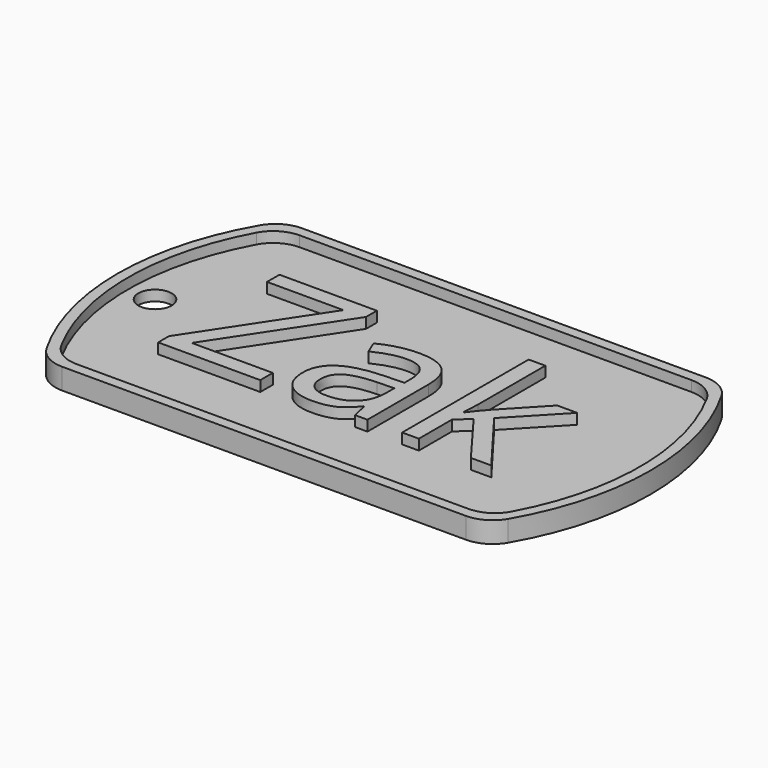
from build123d import *

# Parameters (mm, degrees)
F1_DEPTH     = 1
F3_DEPTH     = 1
F4_R         = 1.5875
F5_DEPTH     = 1
F6_TEXT_SIZE = 19.8251166795
F7_DEPTH     = 1


# Not quite as in the source:
# - a feature of the source that left no trace in its solid (it failed there, or was rolled back) is left out
# - Text() gives the source's letters only with a copy of the font that has no kerning and outlines rounded to 1/6400 em; it was checked with that copy


with BuildPart() as f1:
    # F0 (on Top) → F1 (new body)
    with BuildSketch(Plane.XY):
        with BuildLine():
            ThreePointArc((-19.2474145991, 14.2875), (-20.8349145991, 13.862130657), (-21.9970452561, 12.7))
            ThreePointArc((-21.9970452561, 12.7), (-25.4, 0), (-21.9970452561, -12.7))
            ThreePointArc((-21.9970452561, -12.7), (-20.8349145991, -13.862130657), (-19.2474145991, -14.2875))
            Line((-19.2474145991, -14.2875), (19.2474145991, -14.2875))
            ThreePointArc((19.2474145991, -14.2875), (20.8349145991, -13.862130657), (21.9970452561, -12.7))
            ThreePointArc((21.9970452561, -12.7), (25.4, 0), (21.9970452561, 12.7))
            ThreePointArc((21.9970452561, 12.7), (20.8349145991, 13.862130657), (19.2474145991, 14.2875))
            Line((19.2474145991, 14.2875), (-19.2474145991, 14.2875))
        make_face()
    extrude(amount=F1_DEPTH)

    # F2 (on face) → F3 (join)
    with BuildSketch(Plane.XY.offset(1)):
        with BuildLine():
            Line((19.2474145991, 14.2875), (-19.2474145991, 14.2875))
            ThreePointArc((-19.2474145991, 14.2875), (-20.8349145991, 13.862130657), (-21.9970452561, 12.7))
            ThreePointArc((-21.9970452561, 12.7), (-25.4, 0), (-21.9970452561, -12.7))
            ThreePointArc((-21.9970452561, -12.7), (-20.8349145991, -13.862130657), (-19.2474145991, -14.2875))
            Line((-19.2474145991, -14.2875), (19.2474145991, -14.2875))
            ThreePointArc((19.2474145991, -14.2875), (20.8349145991, -13.862130657), (21.9970452561, -12.7))
            ThreePointArc((21.9970452561, -12.7), (25.4, 0), (21.9970452561, 12.7))
            ThreePointArc((21.9970452561, 12.7), (20.8349145991, 13.862130657), (19.2474145991, 14.2875))
        make_face()
        with BuildLine():
            ThreePointArc((-21.4526124879, 11.6252061249), (-20.2856017842, 12.8404540819), (-18.6611352482, 13.2875))
            Line((-18.6611352482, 13.2875), (18.6611352482, 13.2875))
            ThreePointArc((18.6611352482, 13.2875), (20.2856017842, 12.8404540819), (21.4526124879, 11.6252061249))
            ThreePointArc((21.4526124879, 11.6252061249), (24.4, 0), (21.4526124879, -11.6252061249))
            ThreePointArc((21.4526124879, -11.6252061249), (20.2856017842, -12.8404540819), (18.6611352482, -13.2875))
            Line((18.6611352482, -13.2875), (-18.6611352482, -13.2875))
            ThreePointArc((-18.6611352482, -13.2875), (-20.2856017842, -12.8404540819), (-21.4526124879, -11.6252061249))
            ThreePointArc((-21.4526124879, -11.6252061249), (-24.4, 0), (-21.4526124879, 11.6252061249))
        make_face(mode=Mode.SUBTRACT)
    extrude(amount=F3_DEPTH)

    # F4 (on face) → F5 (cut)
    with BuildSketch(Plane.XY.offset(1)):
        with Locations((-21.821282804, 0)):
            Circle(F4_R)
    extrude(amount=-F5_DEPTH, mode=Mode.SUBTRACT)

    # F6 (on face) → F7 (join)
    with BuildSketch(Plane.XY.offset(1)):
        with Locations((-16.9035214931, -6.761408411)):
            Text('Zak', F6_TEXT_SIZE, font='Open Sans', text_align=(TextAlign.LEFT, TextAlign.BOTTOM))
    extrude(amount=F7_DEPTH)


solid = f1.part
